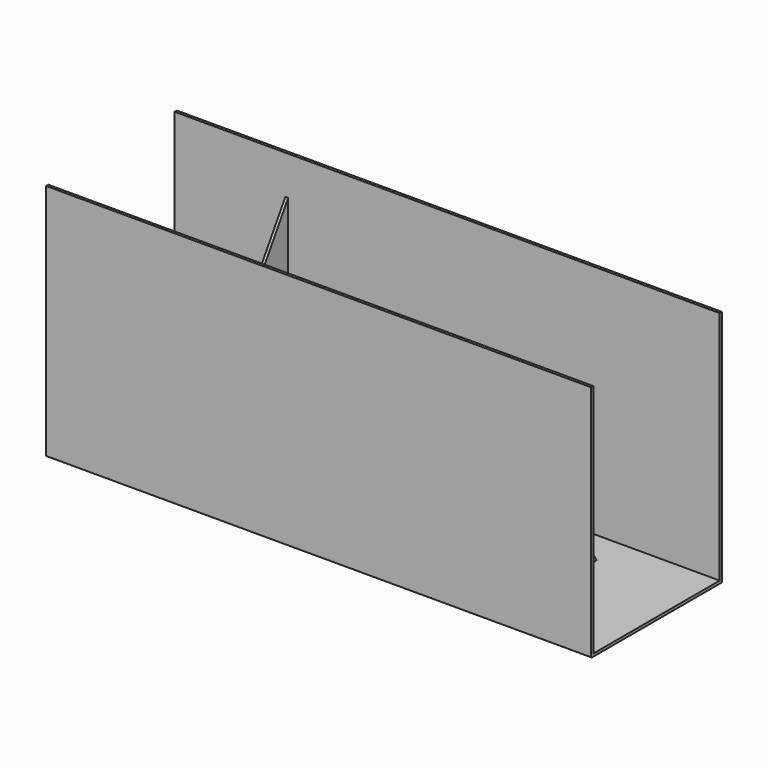
from build123d import *

# Parameters (mm, degrees)
F1_DEPTH = 984
F4_DEPTH = 5
F7_DEPTH = 5
F8_R     = 2


# Not quite as in the source:
# - a feature names something its author has since deleted; it is built from what else it names


with BuildPart() as f1:
    # F0 (on Right) → F1 (new body)
    with BuildSketch(Plane.YZ):
        Polygon((-295, 0), (0, 0), (0, 430), (-5, 430), (-5, 5), (-290, 5), (-290, 430), (-295, 430), align=None)
    extrude(amount=F1_DEPTH)

    # F3 (on offset) → F4 (join)
    with BuildSketch(Plane.YZ.offset(200)):
        Polygon((-230, 0), (-5, 0), (-5, 360), align=None)
    extrude(amount=F4_DEPTH)

    # F6 (on offset) → F7 (join)
    with BuildSketch(Plane.YZ.offset(805)):
        Polygon((-290, 360), (-290, 5), (-65, 5), align=None)
    extrude(amount=F7_DEPTH)

    # F8
    f8_edges = [f1.edges().sort_by_distance(p)[0] for p in [
        (492, 0, 0),
        (492, -295, 0),
    ]]
    fillet(f8_edges, radius=F8_R)


solid = f1.part
